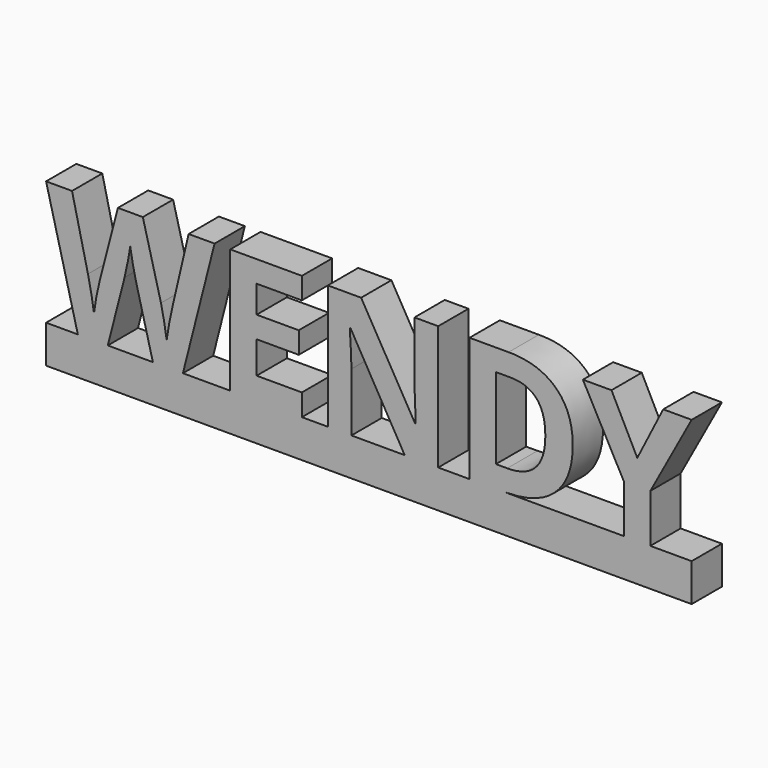
from build123d import *

# Parameters (mm, degrees)
F0_TEXT_SIZE = 46.0507762101
F1_DEPTH     = 10
F2_W         = 170.5821486895
F2_H         = 10
F3_DEPTH     = 10


# Not quite as in the source:
# - Text() gives the source's letters only with a copy of the font that has no kerning and outlines rounded to 1/6400 em; it was checked with that copy


with BuildPart() as f1:
    # F0 (on Front) → F1 (new body)
    with BuildSketch(Plane.XZ):
        with Locations((-74.4983628392, 0)):
            Text('WENDY', F0_TEXT_SIZE, font='Open Sans', font_style=FontStyle.BOLD, text_align=(TextAlign.LEFT, TextAlign.BOTTOM))
    extrude(amount=F1_DEPTH)

    # F2 (on face) → F3 (join)
    with BuildSketch(Plane(origin=(0, 0, 0), x_dir=(1, 0, 0), z_dir=(0, 0, -1))):
        with Locations((10.7927115055, 5)):
            Rectangle(F2_W, F2_H)
    extrude(amount=F3_DEPTH)


solid = f1.part
